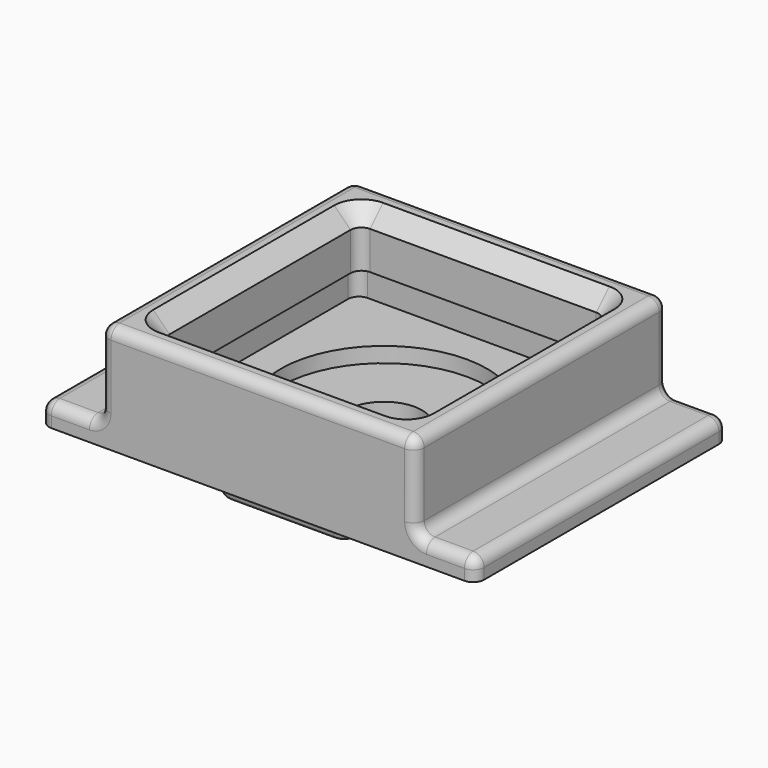
from build123d import *

# Parameters (mm, degrees)
F1_DEPTH  = 2.4
F2_W      = 40
F2_H      = 29
F3_DEPTH  = 2
F4_R      = 9.5
F4_R_2    = 3.5
F5_DEPTH  = 1.4
F6_DEPTH  = 4.4010001
F7_W      = 29
F7_H      = 29
F7_W_2    = 25
F7_H_2    = 25
F8_DEPTH  = 2.9
F9_W      = 29
F9_H      = 29
F9_W_2    = 22.8
F9_H_2    = 22.8
F10_DEPTH = 5
F11_F1_R  = 1
F11_F2_R  = 1
F12_SIZE  = 1.5
F13_R     = 0.5


with BuildPart() as f1:
    # F0 (on Top) → F1 (new body)
    with BuildSketch(Plane.XY):
        with BuildLine():
            Line((0, 11.8), (-4.8, 11.8))
            add(Edge.make_bspline(
                [(-4.8, 11.8), (-5.7190243266, 11.8), (-6.1421032596, 10.873414806), (-6.3, 10)],
                knots=[0, 0, 0, 0, 2.3430749028, 2.3430749028, 2.3430749028, 2.3430749028], degree=3))
            add(Edge.make_bspline(
                [(-6.3, 10), (-6.75, 6.8473730727), (-6.8, 3.4224423006), (-6.8, 0)],
                knots=[0, 0, 0, 0, 10.0124921973, 10.0124921973, 10.0124921973, 10.0124921973], degree=3))
            add(Edge.make_bspline(
                [(-6.3, -10), (-6.75, -6.8473730727), (-6.8, -3.4224423006), (-6.8, 0)],
                knots=[0, 0, 0, 0, 10.0124921973, 10.0124921973, 10.0124921973, 10.0124921973], degree=3))
            add(Edge.make_bspline(
                [(-4.8, -11.8), (-5.7190243266, -11.8), (-6.1421032596, -10.873414806), (-6.3, -10)],
                knots=[0, 0, 0, 0, 2.3430749028, 2.3430749028, 2.3430749028, 2.3430749028], degree=3))
            Line((-4.8, -11.8), (0, -11.8))
            Line((0, -11.8), (4.8, -11.8))
            add(Edge.make_bspline(
                [(4.8, -11.8), (5.7190243266, -11.8), (6.1421032596, -10.873414806), (6.3, -10)],
                knots=[0, 0, 0, 0, 2.3430749028, 2.3430749028, 2.3430749028, 2.3430749028], degree=3))
            add(Edge.make_bspline(
                [(6.3, -10), (6.75, -6.8473730727), (6.8, -3.4224423006), (6.8, 0)],
                knots=[0, 0, 0, 0, 10.0124921973, 10.0124921973, 10.0124921973, 10.0124921973], degree=3))
            add(Edge.make_bspline(
                [(6.3, 10), (6.75, 6.8473730727), (6.8, 3.4224423006), (6.8, 0)],
                knots=[0, 0, 0, 0, 10.0124921973, 10.0124921973, 10.0124921973, 10.0124921973], degree=3))
            add(Edge.make_bspline(
                [(4.8, 11.8), (5.7190243266, 11.8), (6.1421032596, 10.873414806), (6.3, 10)],
                knots=[0, 0, 0, 0, 2.3430749028, 2.3430749028, 2.3430749028, 2.3430749028], degree=3))
            Line((4.8, 11.8), (0, 11.8))
        make_face()
    extrude(amount=F1_DEPTH)

    # F2 (on face) → F3 (join)
    with BuildSketch(Plane.XY.offset(2.4)):
        Rectangle(F2_W, F2_H)
    extrude(amount=F3_DEPTH)

    # F4 (on face) → F5 (cut)
    with BuildSketch(Plane.XY.offset(4.4)):
        Circle(F4_R)
        Circle(F4_R_2, mode=Mode.SUBTRACT)
    extrude(amount=-F5_DEPTH, mode=Mode.SUBTRACT)

    # F6 (cut, through all): a face of the model
    f6_faces = [f1.faces().sort_by_distance(p)[0] for p in [
        (0, 0, 4.4),
    ]]
    extrude(f6_faces, amount=-F6_DEPTH, mode=Mode.SUBTRACT)

    # F7 (on face) → F8 (join)
    with BuildSketch(Plane.XY.offset(4.4)):
        Rectangle(F7_W, F7_H)
        Rectangle(F7_W_2, F7_H_2, mode=Mode.SUBTRACT)
    extrude(amount=F8_DEPTH)

    # F9 (on face) → F10 (join)
    with BuildSketch(Plane.XY.offset(7.3)):
        Rectangle(F9_W, F9_H)
        Rectangle(F9_W_2, F9_H_2, mode=Mode.SUBTRACT)
    extrude(amount=F10_DEPTH)

    # F11: fillet of radius 1 on 24 edges, made by hand

    # F11_f1
    f11_f1_edges = [f1.edges().sort_by_distance(p)[0] for p in [
        (12.5, -12.5, 5.85),
        (11.4, 11.4, 9.8),
        (12.5, 12.5, 5.85),
        (-12.5, -12.5, 5.85),
        (-11.4, -11.4, 9.8),
        (-12.5, 12.5, 5.85),
        (14.5, 0, 4.4),
        (-14.5, 0, 4.4),
        (11.4, -11.4, 9.8),
        (-11.4, 11.4, 9.8),
    ]]
    fillet(f11_f1_edges, radius=F11_F1_R)

    # F11_f2
    f11_f2_edges = [f1.edges().sort_by_distance(p)[0] for p in [
        (-20, -14.5, 3.4),
        (20, -14.5, 3.4),
        (14.5, -14.5, 8.85),
        (-14.5, -14.5, 8.85),
        (-14.5, 14.5, 8.85),
        (-20, 14.5, 3.4),
        (20, 14.5, 3.4),
        (14.5, 14.5, 8.85),
        (-20, 0, 4.4),
        (20, 0, 4.4),
        (14.5, 0, 12.3),
        (0, -14.5, 12.3),
        (-14.5, 0, 12.3),
        (0, 14.5, 12.3),
        (14.7928932188, 14.5, 4.6928932188),
        (-14.7928932188, 14.5, 4.6928932188),
        (-14.7928932188, -14.5, 4.6928932188),
        (14.7928932188, -14.5, 4.6928932188),
    ]]
    fillet(f11_f2_edges, radius=F11_F2_R)

    # F12
    f12_edges = [f1.edges().sort_by_distance(p)[0] for p in [
        (0, 11.4, 12.3),
    ]]
    chamfer(f12_edges, length=F12_SIZE)

    # F13
    f13_edges = [f1.edges().sort_by_distance(p)[0] for p in [
        (-6.722447, -5.009541, 0),
        (0, -11.8, 0),
        (0, 11.8, 0),
        (6.722447, 5.009541, 0),
    ]]
    fillet(f13_edges, radius=F13_R)


solid = f1.part
